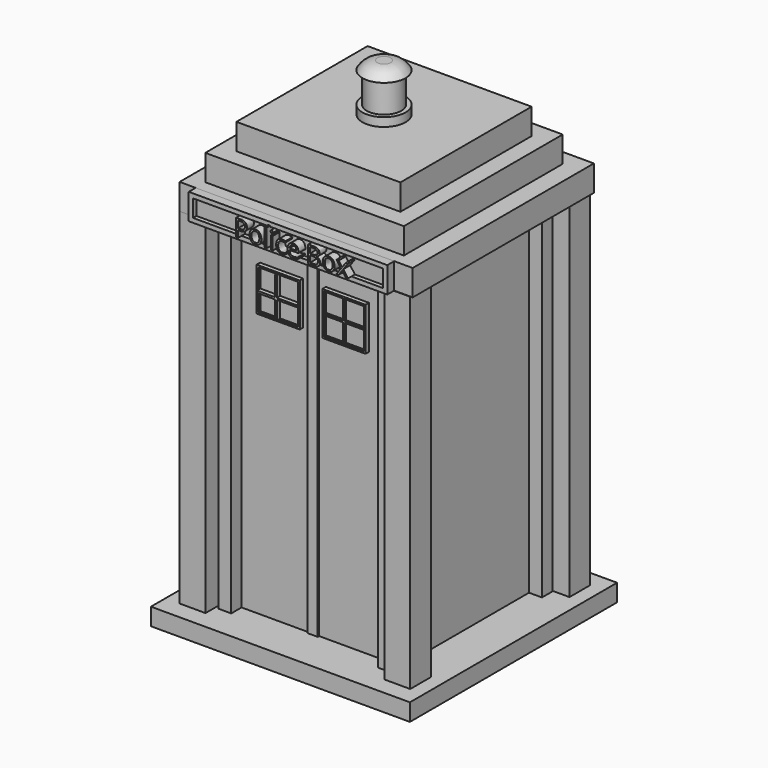
from build123d import *

# Parameters (mm, degrees)
F0_W          = 76.2
F0_H          = 5.08
F1_DEPTH      = 38.1
F1_DEPTH_BACK = 38.1
F2_W          = 50.8
F2_H          = 50.8
F3_DEPTH      = 101.6
F5_W          = 7.62
F5_H          = 7.62
F6_DEPTH      = 101.6
F7_W          = 3.81
F7_H          = 101.6
F8_DEPTH      = 3.81
F9_W          = 3.81
F9_H          = 101.6
F10_DEPTH     = 3.81
F11_W         = 3.81
F11_H         = 101.6
F12_DEPTH     = 3.81
F13_W         = 3.81
F13_H         = 101.6
F14_DEPTH     = 3.81
F15_W         = 12.7
F15_H         = 12.7
F16_DEPTH     = 1.27
F17_T         = -0.508
F17_2_T       = -0.508
F18_W         = 5.2946915091
F18_H         = 0.5755609026
F18_W_2       = 5.842
F18_H_2       = 0.5212312689
F19_DEPTH     = 1.27
F20_W         = 5.3416031877
F20_H         = 0.4991551986
F20_W_2       = 5.842
F21_DEPTH     = 0.508
F22_W         = 3.048
F22_H         = 101.6
F23_DEPTH     = 0.508
F24_W         = 68.58
F24_H         = 66.6492282037
F25_DEPTH     = 7.62
F26_W         = 58.42
F26_H         = 58.42
F27_DEPTH     = 7.62
F28_W         = 48.26
F28_H         = 48.26
F29_DEPTH     = 7.62
F30_R         = 6.35
F31_DEPTH     = 2.54
F32_R         = 5.08
F33_DEPTH     = 8.89
F34_R         = 6.35
F35_DEPTH     = 2.54
F37_W         = 58.42
F37_H         = 7.62
F38_DEPTH     = 2.54
F39_T         = -1.27
F40_TEXT_SIZE = 7.0555555556
F41_DEPTH     = 2.54


# Not quite as in the source:
# - a fillet or chamfer that OpenCascade refuses, or shapes differently, is made with other operations: its cross-section is extruded or revolved along the edge and cut away or added
# - Text() gives the source's letters only with a copy of the font that has no kerning and outlines rounded to 1/6400 em; it was checked with that copy


with BuildPart() as f1:
    # F0 (on Front) → F1 (new body, two sides)
    with BuildSketch(Plane.XZ) as f1_sk:
        Rectangle(F0_W, F0_H)
    extrude(amount=F1_DEPTH)
    extrude(f1_sk.sketch, amount=-F1_DEPTH_BACK)


with BuildPart() as f3:
    # F2 (on face) → F3 (new body)
    with BuildSketch(Plane.XY.offset(2.54)):
        Rectangle(F2_W, F2_H)
    extrude(amount=F3_DEPTH)


with BuildPart() as f6:
    # F5 (on face) → F6 (new body)
    with BuildSketch(Plane.XY.offset(2.54)):
        with Locations((-30.1155748971, -28.9606759325)):
            Rectangle(F5_W, F5_H)
    extrude(amount=F6_DEPTH)


with BuildPart() as f6b:
    # F5 (on face) → F6, piece 2 (new body)
    with BuildSketch(Plane.XY.offset(2.54)):
        with Locations((30.2228812599, 29.4982831454)):
            Rectangle(F5_W, F5_H)
    extrude(amount=F6_DEPTH)


with BuildPart() as f6c:
    # F5 (on face) → F6, piece 3 (new body)
    with BuildSketch(Plane.XY.offset(2.54)):
        with Locations((30.2228812599, -29.0775482082)):
            Rectangle(F5_W, F5_H)
    extrude(amount=F6_DEPTH)


with BuildPart() as f6d:
    # F5 (on face) → F6, piece 4 (new body)
    with BuildSketch(Plane.XY.offset(2.54)):
        with Locations((-29.5684036338, 29.8255219585)):
            Rectangle(F5_W, F5_H)
    extrude(amount=F6_DEPTH)


with BuildPart() as f8:
    # F7 (on face) → F8 (new body)
    with BuildSketch(Plane(origin=(0, 25.4, 0), x_dir=(-1, 0, 0), z_dir=(0, 1, 0))):
        with Locations((-23.495, 53.34)):
            Rectangle(F7_W, F7_H)
    extrude(amount=F8_DEPTH)


with BuildPart() as f8b:
    # F7 (on face) → F8, piece 2 (new body)
    with BuildSketch(Plane(origin=(0, 25.4, 0), x_dir=(-1, 0, 0), z_dir=(0, 1, 0))):
        with Locations((23.495, 53.34)):
            Rectangle(F7_W, F7_H)
    extrude(amount=F8_DEPTH)


with BuildPart() as f10:
    # F9 (on face) → F10 (new body)
    with BuildSketch(Plane.YZ.offset(25.4)):
        with Locations((-23.495, 53.34)):
            Rectangle(F9_W, F9_H)
    extrude(amount=F10_DEPTH)


with BuildPart() as f10b:
    # F9 (on face) → F10, piece 2 (new body)
    with BuildSketch(Plane.YZ.offset(25.4)):
        with Locations((23.495, 53.34)):
            Rectangle(F9_W, F9_H)
    extrude(amount=F10_DEPTH)


with BuildPart() as f12:
    # F11 (on face) → F12 (new body)
    with BuildSketch(Plane.XZ.offset(25.4)):
        with Locations((-23.495, 53.34)):
            Rectangle(F11_W, F11_H)
    extrude(amount=F12_DEPTH)


with BuildPart() as f12b:
    # F11 (on face) → F12, piece 2 (new body)
    with BuildSketch(Plane.XZ.offset(25.4)):
        with Locations((23.495, 53.34)):
            Rectangle(F11_W, F11_H)
    extrude(amount=F12_DEPTH)


with BuildPart() as f14:
    # F13 (on face) → F14 (new body)
    with BuildSketch(Plane(origin=(-25.4, 0, 0), x_dir=(0, -1, 0), z_dir=(-1, 0, 0))):
        with Locations((-23.495, 53.34)):
            Rectangle(F13_W, F13_H)
    extrude(amount=F14_DEPTH)


with BuildPart() as f14b:
    # F13 (on face) → F14, piece 2 (new body)
    with BuildSketch(Plane(origin=(-25.4, 0, 0), x_dir=(0, -1, 0), z_dir=(-1, 0, 0))):
        with Locations((23.495, 53.34)):
            Rectangle(F13_W, F13_H)
    extrude(amount=F14_DEPTH)


with BuildPart() as f16:
    # F15 (on face) → F16 (new body)
    with BuildSketch(Plane.XZ.offset(25.4)):
        with Locations((-9.8032057124, 87.2937029352)):
            Rectangle(F15_W, F15_H)
    extrude(amount=F16_DEPTH)

    # F17
    f17_openings = [f16.faces().sort_by_distance(p)[0] for p in [
        (-9.803206, -26.67, 87.293703),
    ]]
    offset(amount=F17_T, openings=f17_openings)

    # F18 (on face) → F19 (join)
    with BuildSketch(Plane.XZ.offset(25.908)):
        Polygon((-9.8032057124, 93.1357029352), (-10.3505142033, 93.1357029352), (-10.3505142033, 87.2937029352), (-10.3505142033, 86.7181420326), (-10.3505142033, 81.4517029352), (-9.8032057124, 81.4517029352), (-9.8032057124, 86.7724716663), (-9.8032057124, 87.2937029352), align=None)
        with Locations((-12.9978599579, 87.0059224839)):
            Rectangle(F18_W, F18_H)
        with Locations((-6.8822057124, 87.0330873008)):
            Rectangle(F18_W_2, F18_H_2)
    extrude(amount=F19_DEPTH)


with BuildPart() as f16b:
    # F15 (on face) → F16, piece 2 (new body)
    with BuildSketch(Plane.XZ.offset(25.4)):
        with Locations((9.549175376, 87.2937029352)):
            Rectangle(F15_W, F15_H)
    extrude(amount=F16_DEPTH)

    # F17#2
    f17_2_openings = [f16b.faces().sort_by_distance(p)[0] for p in [
        (9.549175, -26.67, 87.293703),
    ]]
    offset(amount=F17_2_T, openings=f17_2_openings)

    # F20 (on face) → F21 (join)
    with BuildSketch(Plane.XZ.offset(25.908)):
        Polygon((9.549175376, 93.1357029352), (9.0487785637, 93.1357029352), (9.0487785637, 87.2937029352), (9.0487785637, 86.7945477366), (9.0487785637, 81.4517029352), (9.549175376, 81.4517029352), (9.549175376, 86.7945477366), (9.549175376, 87.2937029352), align=None)
        with Locations((6.3779769699, 87.0441253359)):
            Rectangle(F20_W, F20_H)
        with Locations((12.470175376, 87.0441253359)):
            Rectangle(F20_W_2, F20_H)
    extrude(amount=F21_DEPTH)


with BuildPart() as f23:
    # F22 (on face) → F23 (new body)
    with BuildSketch(Plane.XZ.offset(25.4)):
        with Locations((-0.3089322338, 53.34)):
            Rectangle(F22_W, F22_H)
    extrude(amount=F23_DEPTH)


with BuildPart() as f25:
    # F24 (on face) → F25 (new body)
    with BuildSketch(Plane.XY.offset(104.14)):
        with Locations((0.3644251029, 0.5539381694)):
            Rectangle(F24_W, F24_H)
    extrude(amount=F25_DEPTH)

    # F26 (on face) → F27 (join)
    with BuildSketch(Plane.XY.offset(111.76)):
        Rectangle(F26_W, F26_H)
    extrude(amount=F27_DEPTH)

    # F28 (on face) → F29 (join)
    with BuildSketch(Plane.XY.offset(119.38)):
        Rectangle(F28_W, F28_H)
    extrude(amount=F29_DEPTH)

    # F30 (on face) → F31 (join)
    with BuildSketch(Plane.XY.offset(127)):
        Circle(F30_R)
    extrude(amount=F31_DEPTH)


with BuildPart() as f33:
    # F32 (on face) → F33 (new body)
    with BuildSketch(Plane.XY.offset(129.54)):
        Circle(F32_R)
    extrude(amount=F33_DEPTH)


with BuildPart() as f35:
    # F34 (on face) → F35 (new body)
    with BuildSketch(Plane.XY.offset(138.43)):
        Circle(F34_R)
    extrude(amount=F35_DEPTH)

    # F36: fillet of radius 5.08 on 1 edges, made by hand

    # F36_s1 → F36_t2 (revolve, cut)
    with BuildSketch(Plane.XZ):
        with BuildLine():
            ThreePointArc((6.35, 138.43), (4.4905909488, 140.2894090512), (1.9505909488, 140.97))
            Line((1.9505909488, 140.97), (6.35, 140.97))
            Line((6.35, 140.97), (6.35, 138.43))
        make_face()
    revolve(axis=Axis((0, 0, 140.97), (0, 0, 1)), mode=Mode.SUBTRACT)


with BuildPart() as f38:
    # F37 (on face) → F38 (new body)
    with BuildSketch(Plane.XZ.offset(32.7706759325)):
        with Locations((0, 107.95)):
            Rectangle(F37_W, F37_H)
    extrude(amount=F38_DEPTH)

    # F39
    f39_openings = [f38.faces().sort_by_distance(p)[0] for p in [
        (0, -35.310676, 107.95),
    ]]
    offset(amount=F39_T, openings=f39_openings)


with BuildPart() as f41:
    # F40 (on face) → F41 (new body)
    with BuildSketch(Plane.XZ.offset(34.0406759325)):
        with Locations((-14.9514852092, 105.41)):
            Text('Police Box', F40_TEXT_SIZE, font='Open Sans', text_align=(TextAlign.LEFT, TextAlign.BOTTOM))
    extrude(amount=F41_DEPTH)


solid = Compound([f1.part, f3.part, f6.part, f6b.part, f6c.part, f6d.part, f8.part, f8b.part, f10.part, f10b.part, f12.part, f12b.part, f14.part, f14b.part, f16.part, f16b.part, f23.part, f25.part, f33.part, f35.part, f38.part, f41.part])
